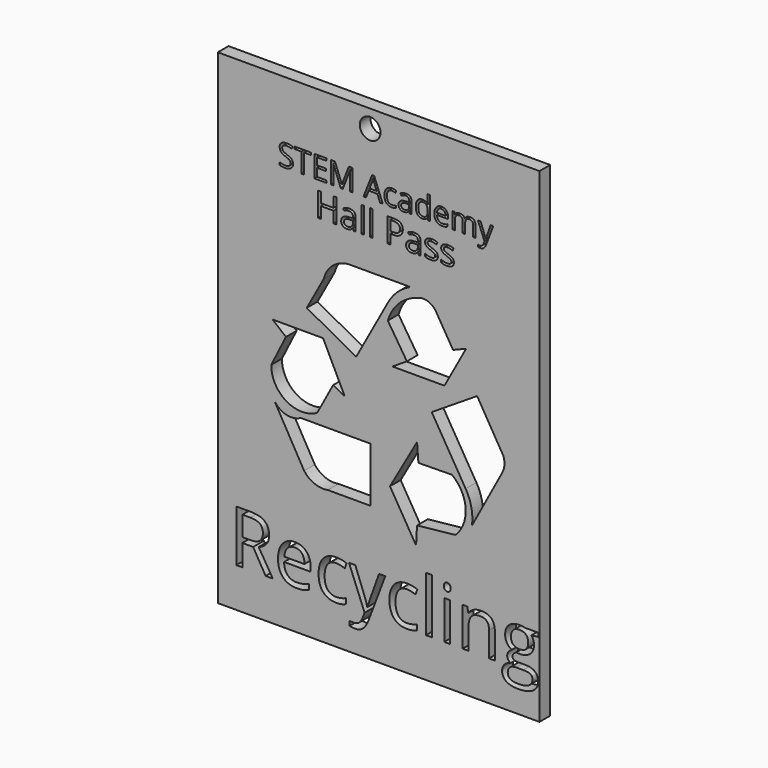
from build123d import *

# Parameters (mm, degrees)
F0_W           = 76.2
F0_H           = 114.8772763218
F1_DEPTH       = 3.175
F2_R           = 2.4570796673
F2_TEXT_SIZE   = 7.1951446848
F2_TEXT_SIZE_2 = 7.9946023309
F2_TEXT_SIZE_3 = 17.1255475531
F3_DEPTH       = 3.175


# Not quite as in the source:
# - Text() gives the source's letters only with a copy of the font that has no kerning and outlines rounded to 1/6400 em; it was checked with that copy


with BuildPart() as f1:
    # F0 (on Front) → F1 (new body)
    with BuildSketch(Plane.XZ):
        with Locations((8.0585610121, 10.6488130987)):
            Rectangle(F0_W, F0_H)
    extrude(amount=F1_DEPTH)

    # F2 (on face) → F3 (cut)
    with BuildSketch(Plane.XZ.offset(3.175)):
        with BuildLine():
            Line((-4.9126631824, 29.0469050428), (-8.9670447633, 21.630352363))
            Line((-8.9670447633, 21.630352363), (2.7384413406, 15.2313541621))
            Line((2.7384413406, 15.2313541621), (10.2909414628, 29.0469050428))
            ThreePointArc((10.2909414628, 29.0469050428), (12.5199980609, 31.9238363289), (15.5364396051, 33.960133791))
            Line((15.5364396051, 33.960133791), (1.3337832643, 33.960133791))
            ThreePointArc((1.3337832643, 33.960133791), (-2.6398142853, 32.58464508), (-4.9126631824, 29.0469050428))
        make_face()
        with BuildLine():
            Line((14.7560741752, 18.1967429817), (11.3224638626, 16.0117186606))
            Line((11.3224638626, 16.0117186606), (23.6522443593, 16.0117186606))
            Line((23.6522443593, 16.0117186606), (28.7786257047, 25.3892467859))
            Line((28.7786257047, 25.3892467859), (25.6811957806, 24.1275243461))
            Line((25.6811957806, 24.1275243461), (21.6232910752, 30.8386683464))
            ThreePointArc((21.6232910752, 30.8386683464), (19.7010099107, 32.358417544), (17.2532442957, 32.2433263063))
            ThreePointArc((17.2532442957, 32.2433263063), (12.841360991, 29.6319179487), (10.2299526334, 25.220034644))
            Line((10.2299526334, 25.220034644), (14.7560741752, 18.1967429817))
        make_face()
        with BuildLine():
            Line((6.1720511876, -1.7806198448), (-10.3717036545, -1.7806198448))
            ThreePointArc((-10.3717036545, -1.7806198448), (-13.9370455338, -2.205035966), (-16.7707018554, 0))
            Line((-16.7707018554, 0), (-9.5913372934, -12.5496657565))
            ThreePointArc((-9.5913372934, -12.5496657565), (-7.0927166228, -14.4411105004), (-3.9727040567, -14.7346919402))
            Line((-3.9727040567, -14.7346919402), (6.1720511876, -14.7346919402))
            Line((6.1720511876, -14.7346919402), (6.1720511876, -1.7806198448))
        make_face()
        with BuildLine():
            Line((-13.9070646837, 13.9686986804), (-17.3854269087, 7.0154429413))
            ThreePointArc((-17.3854269087, 7.0154429413), (-13.8357570007, 0.6230490929), (-6.5249381587, 0.5014619674))
            Line((-6.5249381587, 0.5014619674), (-2.720661927, 7.5634522364))
            Line((-2.720661927, 7.5634522364), (0, 6.1524263583))
            Line((0, 6.1524263583), (-5.1074833609, 16.5746882558))
            Line((-5.1074833609, 16.5746882558), (-17.0563682914, 16.5746882558))
            Line((-17.0563682914, 16.5746882558), (-13.9070646837, 13.9686986804))
        make_face()
        with BuildLine():
            Line((20.6346958876, 9.5264967531), (28.6686196923, -3.8318971638))
            ThreePointArc((28.6686196923, -3.8318971638), (30.0297166676, -7.288835349), (30.1870070398, -11.0007440671))
            Line((30.1870070398, -11.0007440671), (37.3608022928, 2.3627064656))
            ThreePointArc((37.3608022928, 2.3627064656), (37.8631320151, 4.1311260929), (37.5792458653, 5.9474552982))
            Line((37.5792458653, 5.9474552982), (31.3910022378, 16.3735449314))
            Line((31.3910022378, 16.3735449314), (20.6346958876, 9.5264967531))
        make_face()
        with BuildLine():
            ThreePointArc((26.2753646821, -14.2608406022), (28.6713535845, -7.9242761595), (25.4104342312, -1.9863289781))
            Line((25.4104342312, -1.9863289781), (17.4806620926, -2.0975924563))
            Line((17.4806620926, -2.0975924563), (17.1561911702, 2.1387347952))
            Line((17.1561911702, 2.1387347952), (10.7434671372, -9.1605586931))
            Line((10.7434671372, -9.1605586931), (16.9317498803, -19.4780211896))
            Line((16.9317498803, -19.4780211896), (17.1504113823, -15.2415139601))
            Line((17.1504113823, -15.2415139601), (26.2753646821, -14.2608406022))
        make_face()
        with Locations((6.0439212248, 63.892878592)):
            Circle(F2_R)
        with Locations((-15.8293172717, 49.2147877812)):
            Text('STEM Academy', F2_TEXT_SIZE, font='Open Sans', text_align=(TextAlign.LEFT, TextAlign.BOTTOM))
        with Locations((-7.0809904719, 41.2738025188)):
            Text('Hall Pass', F2_TEXT_SIZE_2, font='Open Sans', text_align=(TextAlign.LEFT, TextAlign.BOTTOM))
        with Locations((-27.3278570385, -37.4379679561)):
            Text('Recycling', F2_TEXT_SIZE_3, font='Open Sans', text_align=(TextAlign.LEFT, TextAlign.BOTTOM))
    extrude(amount=-F3_DEPTH, mode=Mode.SUBTRACT)


solid = f1.part
